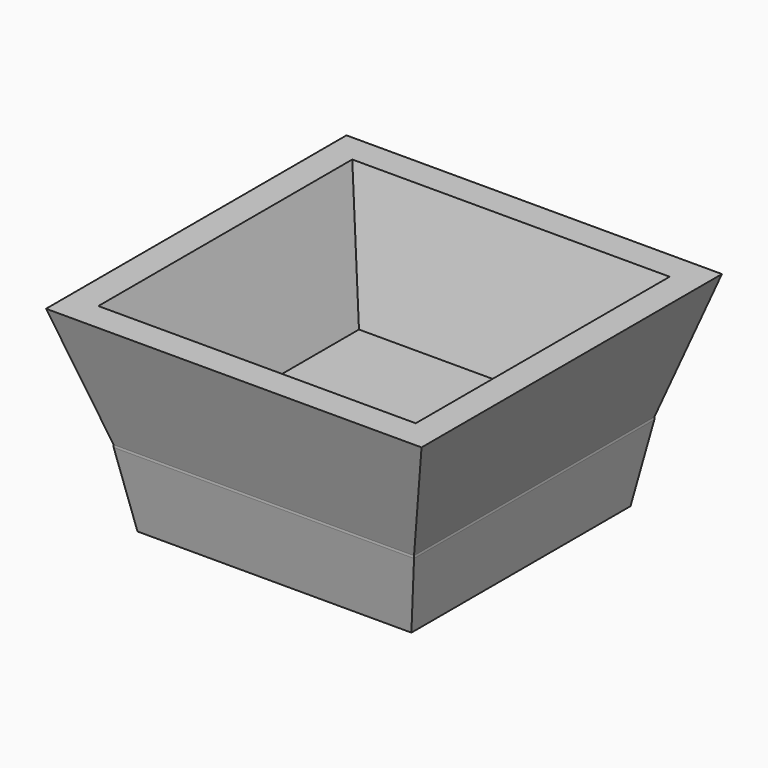
from build123d import *

# Parameters (mm, degrees)
F0_W          = 19.05
F0_H          = 19.05
F0_W_2        = 12.7
F0_H_2        = 12.7
F1_DEPTH      = 6.35
F2_W          = 15.24
F2_H          = 15.24
F3_DEPTH      = 3.81
F4_SIZE2      = 6.34999
F4_SIZE       = 1.701467
F5_T4_DEPTH   = 52.0165982025
F5_T10_DEPTH  = 52.0165982025
F5_T16_DEPTH  = 52.0165982025
F5_T23_DEPTH  = 52.0165982025
F5_T29_DEPTH  = 52.0165982025
F5_T35_DEPTH  = 52.0165982025
F5_T41_DEPTH  = 52.0165982025
F5_T47_DEPTH  = 52.0165982025
F5_T54_DEPTH  = 52.0165982025
F5_T60_DEPTH  = 52.0165982025
F5_T66_DEPTH  = 52.0165982025
F5_T72_DEPTH  = 52.0165982025
F5_T78_DEPTH  = 52.0165982025
F5_T85_DEPTH  = 52.0165982025
F5_T91_DEPTH  = 52.0165982025
F5_T97_DEPTH  = 52.0165982025
F5_T103_DEPTH = 52.0165982025
F5_T109_DEPTH = 52.0165982025
F5_T116_DEPTH = 52.0165982025
F5_T122_DEPTH = 52.0165982025
F6_C1_SIZE2   = 0.6718057965
F6_C1_SIZE    = 3.81
F6_C2_SIZE2   = 0.6718057965
F6_C2_SIZE    = 3.81
F6_C3_SIZE2   = 3.81
F6_C3_SIZE    = 0.6718057965
F6_C4_SIZE2   = 3.81
F6_C4_SIZE    = 0.6718057965


# Not quite as in the source:
# - a fillet or chamfer that OpenCascade refuses, or shapes differently, is made with other operations: its cross-section is extruded or revolved along the edge and cut away or added
# - a fillet or chamfer is up to 0.001 mm smaller than in the source, because OpenCascade refuses the exact size


with BuildPart() as f1:
    # F0 (on Top) → F1 (new body)
    with BuildSketch(Plane.XY):
        Rectangle(F0_W, F0_H)
        Rectangle(F0_W_2, F0_H_2, mode=Mode.SUBTRACT)
    extrude(amount=F1_DEPTH)

    # F2 (on Top) → F3 (join)
    with BuildSketch(Plane.XY):
        Rectangle(F2_W, F2_H)
    extrude(amount=-F3_DEPTH)

    # F4 (size 1.7014773719 and 6.35 in the source; OpenCascade refuses exactly that, so slightly less here)
    f4_edges = [f1.edges().sort_by_distance(p)[0] for p in [
        (0, 6.35, 6.35),
        (6.35, 0, 6.35),
        (0, -6.35, 6.35),
        (-6.35, 0, 6.35),
    ]]
    f4_side = f1.faces().sort_by_distance((9.255592, 0, 6.35))[0]
    chamfer(f4_edges, length=F4_SIZE, length2=F4_SIZE2, reference=f4_side)

    # F5: chamfer of 6.35 x 1.9413898273 on 4 edges, made by hand


with BuildPart() as f5_tool2:
    # F5_s3 → F5_t4 (new body)
    with BuildSketch(Plane.YZ.offset(26.0082991012)):
        Polygon((9.525, 6.35), (7.5836101727, 0), (9.525, 0), align=None)
    extrude(amount=-F5_T4_DEPTH)

    split(bisect_by=Plane.XZ.offset(-7.62), keep=Keep.BOTTOM)

    split(bisect_by=Plane.YZ.offset(7.62), keep=Keep.TOP)


with BuildPart() as f1_1:
    add(f1.part)

    # F5_t1: cut F5_tool2
    add(f5_tool2.part, mode=Mode.SUBTRACT)


with BuildPart() as f5_tool8:
    # F5_s9 → F5_t10 (new body)
    with BuildSketch(Plane.YZ.offset(26.0082991012)):
        Polygon((9.525, 6.35), (7.5836101727, 0), (9.525, 0), align=None)
    extrude(amount=-F5_T10_DEPTH)

    split(bisect_by=Plane.XZ.offset(-7.62), keep=Keep.TOP)

    split(bisect_by=Plane.YZ.offset(7.62), keep=Keep.TOP)


with BuildPart() as f1_2:
    add(f1_1.part)

    # F5_t7: cut F5_tool8
    add(f5_tool8.part, mode=Mode.SUBTRACT)


with BuildPart() as f5_tool14:
    # F5_s15 → F5_t16 (new body)
    with BuildSketch(Plane.YZ.offset(26.0082991012)):
        Polygon((9.525, 6.35), (7.5836101727, 0), (9.525, 0), align=None)
    extrude(amount=-F5_T16_DEPTH)

    split(bisect_by=Plane.XZ.offset(-7.62), keep=Keep.BOTTOM)

    split(bisect_by=Plane.YZ.offset(-7.62), keep=Keep.TOP)

    split(bisect_by=Plane.YZ.offset(7.62), keep=Keep.BOTTOM)


with BuildPart() as f1_3:
    add(f1_2.part)

    # F5_t13: cut F5_tool14
    add(f5_tool14.part, mode=Mode.SUBTRACT)


with BuildPart() as f5_tool21:
    # F5_s22 → F5_t23 (new body)
    with BuildSketch(Plane.YZ.offset(26.0082991012)):
        Polygon((9.525, 6.35), (7.5836101727, 0), (9.525, 0), align=None)
    extrude(amount=-F5_T23_DEPTH)

    split(bisect_by=Plane.XZ.offset(-7.62), keep=Keep.BOTTOM)

    split(bisect_by=Plane.YZ.offset(-7.62), keep=Keep.BOTTOM)


with BuildPart() as f1_4:
    add(f1_3.part)

    # F5_t20: cut F5_tool21
    add(f5_tool21.part, mode=Mode.SUBTRACT)


with BuildPart() as f5_tool27:
    # F5_s28 → F5_t29 (new body)
    with BuildSketch(Plane.YZ.offset(26.0082991012)):
        Polygon((9.525, 6.35), (7.5836101727, 0), (9.525, 0), align=None)
    extrude(amount=-F5_T29_DEPTH)

    split(bisect_by=Plane.XZ.offset(-7.62), keep=Keep.TOP)

    split(bisect_by=Plane.YZ.offset(-7.62), keep=Keep.BOTTOM)


with BuildPart() as f1_5:
    add(f1_4.part)

    # F5_t26: cut F5_tool27
    add(f5_tool27.part, mode=Mode.SUBTRACT)


with BuildPart() as f5_tool33:
    # F5_s34 → F5_t35 (new body)
    with BuildSketch(Plane.XZ.offset(26.0082991012)):
        Polygon((9.525, 6.35), (7.5836101727, 0), (9.525, 0), align=None)
    extrude(amount=-F5_T35_DEPTH)

    split(bisect_by=Plane.XZ.offset(7.62), keep=Keep.TOP)

    split(bisect_by=Plane.YZ.offset(7.62), keep=Keep.TOP)


with BuildPart() as f1_6:
    add(f1_5.part)

    # F5_t32: cut F5_tool33
    add(f5_tool33.part, mode=Mode.SUBTRACT)


with BuildPart() as f5_tool39:
    # F5_s40 → F5_t41 (new body)
    with BuildSketch(Plane.XZ.offset(26.0082991012)):
        Polygon((9.525, 6.35), (7.5836101727, 0), (9.525, 0), align=None)
    extrude(amount=-F5_T41_DEPTH)

    split(bisect_by=Plane.XZ.offset(7.62), keep=Keep.TOP)

    split(bisect_by=Plane.YZ.offset(7.62), keep=Keep.BOTTOM)


with BuildPart() as f1_7:
    add(f1_6.part)

    # F5_t38: cut F5_tool39
    add(f5_tool39.part, mode=Mode.SUBTRACT)


with BuildPart() as f5_tool45:
    # F5_s46 → F5_t47 (new body)
    with BuildSketch(Plane.XZ.offset(26.0082991012)):
        Polygon((9.525, 6.35), (7.5836101727, 0), (9.525, 0), align=None)
    extrude(amount=-F5_T47_DEPTH)

    split(bisect_by=Plane.XZ.offset(-7.62), keep=Keep.TOP)

    split(bisect_by=Plane.XZ.offset(7.62), keep=Keep.BOTTOM)

    split(bisect_by=Plane.YZ.offset(7.62), keep=Keep.TOP)


with BuildPart() as f1_8:
    add(f1_7.part)

    # F5_t44: cut F5_tool45
    add(f5_tool45.part, mode=Mode.SUBTRACT)


with BuildPart() as f5_tool52:
    # F5_s53 → F5_t54 (new body)
    with BuildSketch(Plane.XZ.offset(26.0082991012)):
        Polygon((9.525, 6.35), (7.5836101727, 0), (9.525, 0), align=None)
    extrude(amount=-F5_T54_DEPTH)

    split(bisect_by=Plane.XZ.offset(-7.62), keep=Keep.BOTTOM)

    split(bisect_by=Plane.YZ.offset(7.62), keep=Keep.TOP)


with BuildPart() as f1_9:
    add(f1_8.part)

    # F5_t51: cut F5_tool52
    add(f5_tool52.part, mode=Mode.SUBTRACT)


with BuildPart() as f5_tool58:
    # F5_s59 → F5_t60 (new body)
    with BuildSketch(Plane.XZ.offset(26.0082991012)):
        Polygon((9.525, 6.35), (7.5836101727, 0), (9.525, 0), align=None)
    extrude(amount=-F5_T60_DEPTH)

    split(bisect_by=Plane.XZ.offset(-7.62), keep=Keep.BOTTOM)

    split(bisect_by=Plane.YZ.offset(7.62), keep=Keep.BOTTOM)


with BuildPart() as f1_10:
    add(f1_9.part)

    # F5_t57: cut F5_tool58
    add(f5_tool58.part, mode=Mode.SUBTRACT)


with BuildPart() as f5_tool64:
    # F5_s65 → F5_t66 (new body)
    with BuildSketch(Plane.YZ.offset(-26.0082991012)):
        Polygon((-9.525, 6.35), (-7.5836101727, 0), (-9.525, 0), align=None)
    extrude(amount=F5_T66_DEPTH)

    split(bisect_by=Plane.YZ.offset(-7.62), keep=Keep.BOTTOM)

    split(bisect_by=Plane.XZ.offset(7.62), keep=Keep.TOP)


with BuildPart() as f1_11:
    add(f1_10.part)

    # F5_t63: cut F5_tool64
    add(f5_tool64.part, mode=Mode.SUBTRACT)


with BuildPart() as f5_tool70:
    # F5_s71 → F5_t72 (new body)
    with BuildSketch(Plane.YZ.offset(-26.0082991012)):
        Polygon((-9.525, 6.35), (-7.5836101727, 0), (-9.525, 0), align=None)
    extrude(amount=F5_T72_DEPTH)

    split(bisect_by=Plane.YZ.offset(-7.62), keep=Keep.BOTTOM)

    split(bisect_by=Plane.XZ.offset(7.62), keep=Keep.BOTTOM)


with BuildPart() as f1_12:
    add(f1_11.part)

    # F5_t69: cut F5_tool70
    add(f5_tool70.part, mode=Mode.SUBTRACT)


with BuildPart() as f5_tool76:
    # F5_s77 → F5_t78 (new body)
    with BuildSketch(Plane.YZ.offset(-26.0082991012)):
        Polygon((-9.525, 6.35), (-7.5836101727, 0), (-9.525, 0), align=None)
    extrude(amount=F5_T78_DEPTH)

    split(bisect_by=Plane.YZ.offset(-7.62), keep=Keep.TOP)

    split(bisect_by=Plane.XZ.offset(7.62), keep=Keep.TOP)

    split(bisect_by=Plane.YZ.offset(7.62), keep=Keep.BOTTOM)


with BuildPart() as f1_13:
    add(f1_12.part)

    # F5_t75: cut F5_tool76
    add(f5_tool76.part, mode=Mode.SUBTRACT)


with BuildPart() as f5_tool83:
    # F5_s84 → F5_t85 (new body)
    with BuildSketch(Plane.YZ.offset(-26.0082991012)):
        Polygon((-9.525, 6.35), (-7.5836101727, 0), (-9.525, 0), align=None)
    extrude(amount=F5_T85_DEPTH)

    split(bisect_by=Plane.XZ.offset(7.62), keep=Keep.TOP)

    split(bisect_by=Plane.YZ.offset(7.62), keep=Keep.TOP)


with BuildPart() as f1_14:
    add(f1_13.part)

    # F5_t82: cut F5_tool83
    add(f5_tool83.part, mode=Mode.SUBTRACT)


with BuildPart() as f5_tool89:
    # F5_s90 → F5_t91 (new body)
    with BuildSketch(Plane.YZ.offset(-26.0082991012)):
        Polygon((-9.525, 6.35), (-7.5836101727, 0), (-9.525, 0), align=None)
    extrude(amount=F5_T91_DEPTH)

    split(bisect_by=Plane.XZ.offset(7.62), keep=Keep.BOTTOM)

    split(bisect_by=Plane.YZ.offset(7.62), keep=Keep.TOP)


with BuildPart() as f1_15:
    add(f1_14.part)

    # F5_t88: cut F5_tool89
    add(f5_tool89.part, mode=Mode.SUBTRACT)


with BuildPart() as f5_tool95:
    # F5_s96 → F5_t97 (new body)
    with BuildSketch(Plane.XZ.offset(-26.0082991012)):
        Polygon((-9.525, 6.35), (-7.5836101727, 0), (-9.525, 0), align=None)
    extrude(amount=F5_T97_DEPTH)

    split(bisect_by=Plane.XZ.offset(-7.62), keep=Keep.BOTTOM)

    split(bisect_by=Plane.YZ.offset(-7.62), keep=Keep.BOTTOM)


with BuildPart() as f1_16:
    add(f1_15.part)

    # F5_t94: cut F5_tool95
    add(f5_tool95.part, mode=Mode.SUBTRACT)


with BuildPart() as f5_tool101:
    # F5_s102 → F5_t103 (new body)
    with BuildSketch(Plane.XZ.offset(-26.0082991012)):
        Polygon((-9.525, 6.35), (-7.5836101727, 0), (-9.525, 0), align=None)
    extrude(amount=F5_T103_DEPTH)

    split(bisect_by=Plane.XZ.offset(-7.62), keep=Keep.BOTTOM)

    split(bisect_by=Plane.YZ.offset(-7.62), keep=Keep.TOP)


with BuildPart() as f1_17:
    add(f1_16.part)

    # F5_t100: cut F5_tool101
    add(f5_tool101.part, mode=Mode.SUBTRACT)


with BuildPart() as f5_tool107:
    # F5_s108 → F5_t109 (new body)
    with BuildSketch(Plane.XZ.offset(-26.0082991012)):
        Polygon((-9.525, 6.35), (-7.5836101727, 0), (-9.525, 0), align=None)
    extrude(amount=F5_T109_DEPTH)

    split(bisect_by=Plane.XZ.offset(-7.62), keep=Keep.TOP)

    split(bisect_by=Plane.YZ.offset(-7.62), keep=Keep.BOTTOM)

    split(bisect_by=Plane.XZ.offset(7.62), keep=Keep.BOTTOM)


with BuildPart() as f1_18:
    add(f1_17.part)

    # F5_t106: cut F5_tool107
    add(f5_tool107.part, mode=Mode.SUBTRACT)


with BuildPart() as f5_tool114:
    # F5_s115 → F5_t116 (new body)
    with BuildSketch(Plane.XZ.offset(-26.0082991012)):
        Polygon((-9.525, 6.35), (-7.5836101727, 0), (-9.525, 0), align=None)
    extrude(amount=F5_T116_DEPTH)

    split(bisect_by=Plane.YZ.offset(-7.62), keep=Keep.BOTTOM)

    split(bisect_by=Plane.XZ.offset(7.62), keep=Keep.TOP)


with BuildPart() as f1_19:
    add(f1_18.part)

    # F5_t113: cut F5_tool114
    add(f5_tool114.part, mode=Mode.SUBTRACT)


with BuildPart() as f5_tool120:
    # F5_s121 → F5_t122 (new body)
    with BuildSketch(Plane.XZ.offset(-26.0082991012)):
        Polygon((-9.525, 6.35), (-7.5836101727, 0), (-9.525, 0), align=None)
    extrude(amount=F5_T122_DEPTH)

    split(bisect_by=Plane.YZ.offset(-7.62), keep=Keep.TOP)

    split(bisect_by=Plane.XZ.offset(7.62), keep=Keep.TOP)


with BuildPart() as f1_20:
    add(f1_19.part)

    # F5_t119: cut F5_tool120
    add(f5_tool120.part, mode=Mode.SUBTRACT)

    # F6: chamfer of 3.81 x 0.6718057965 on 4 edges, made by hand

    # F6_c1
    f6_c1_edges = [f1_20.edges().sort_by_distance(p)[0] for p in [
        (0, -7.62, -3.81),
    ]]
    f6_c1_side = f1_20.faces().sort_by_distance((0, -7.62, -3.7965638841))[0]
    chamfer(f6_c1_edges, length=F6_C1_SIZE, length2=F6_C1_SIZE2, reference=f6_c1_side)

    # F6_c2
    f6_c2_edges = [f1_20.edges().sort_by_distance(p)[0] for p in [
        (7.62, 0.3359028982, -3.81),
    ]]
    f6_c2_side = f1_20.faces().sort_by_distance((7.62, 0.3359028982, -3.7965638841))[0]
    chamfer(f6_c2_edges, length=F6_C2_SIZE, length2=F6_C2_SIZE2, reference=f6_c2_side)

    # F6_c3
    f6_c3_edges = [f1_20.edges().sort_by_distance(p)[0] for p in [
        (-0.3359028982, 7.62, -3.81),
    ]]
    f6_c3_side = f1_20.faces().sort_by_distance((-0.3359028982, 7.6065638841, -3.81))[0]
    chamfer(f6_c3_edges, length=F6_C3_SIZE, length2=F6_C3_SIZE2, reference=f6_c3_side)

    # F6_c4
    f6_c4_edges = [f1_20.edges().sort_by_distance(p)[0] for p in [
        (-7.62, 0, -3.81),
    ]]
    f6_c4_side = f1_20.faces().sort_by_distance((-7.6065638841, 0, -3.81))[0]
    chamfer(f6_c4_edges, length=F6_C4_SIZE, length2=F6_C4_SIZE2, reference=f6_c4_side)


solid = f1_20.part
